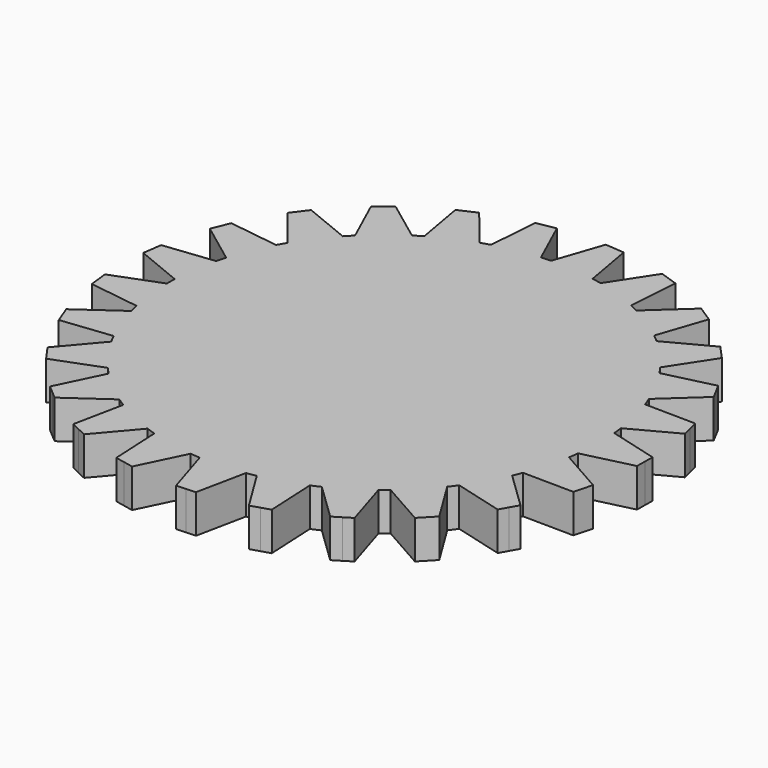
from build123d import *

# Parameters (mm, degrees)
F1_DEPTH = 4


# Not quite as in the source:
# - a feature names something its author has since deleted; it is built from what else it names


with BuildPart() as f1:
    # F0 (on Top) → F1 (new body)
    with BuildSketch(Plane.XY):
        with BuildLine():
            ThreePointArc((-15.8207142224, 15.9985937349), (-16.1763177404, 15.6389495927), (-16.5237476958, 15.2714034091))
            ThreePointArc((-16.5237476958, 15.2714034091), (-17.2896362976, 14.3985581465), (-18.0094723367, 13.4873609781))
            ThreePointArc((-18.0094723367, 13.4873609781), (-18.6807530995, 12.5411109411), (-19.3023658635, 11.5615168585))
            ThreePointArc((-19.3023658635, 11.5615168585), (-19.557357582, 11.1247365996), (-19.8024673676, 10.6823352389))
            ThreePointArc((-19.8024673676, 10.6823352389), (-20.7974411865, 8.585827863), (-21.5711788684, 6.3979873576))
            ThreePointArc((-21.5711788684, 6.3979873576), (-21.7095367198, 5.9115154921), (-21.8369251863, 5.4220566587))
            ThreePointArc((-21.8369251863, 5.4220566587), (-22.2792598903, 3.1439749905), (-22.4845953717, 0.8324487809))
            ThreePointArc((-22.4845953717, 0.8324487809), (-22.4976258234, 0.3268521252), (-22.4992886849, -0.1789096823))
            ThreePointArc((-22.4992886849, -0.1789096823), (-22.3611907578, -2.4954253934), (-21.9852220552, -4.7853956142))
            ThreePointArc((-21.9852220552, -4.7853956142), (-21.872106356, -5.2783485629), (-21.7479391288, -5.76863447))
            ThreePointArc((-21.7479391288, -5.76863447), (-21.0380857712, -7.9780290224), (-20.104436381, -10.1025560035))
            ThreePointArc((-20.104436381, -10.1025560035), (-19.8722820063, -10.5518911983), (-19.630086574, -10.9958947383))
            ThreePointArc((-19.630086574, -10.9958947383), (-18.393080483, -12.9593437467), (-16.96041503, -14.7849356444))
            ThreePointArc((-16.96041503, -14.7849356444), (-16.623809093, -15.1624197026), (-16.2788034853, -15.5322425002))
            ThreePointArc((-16.2788034853, -15.5322425002), (-14.5923703031, -17.1263752422), (-12.7507084267, -18.5383234036))
            ThreePointArc((-12.7507084267, -18.5383234036), (-12.3308011164, -18.8202376135), (-11.9046633044, -19.0926423422))
            ThreePointArc((-11.9046633044, -19.0926423422), (-9.87476783, -20.2172935949), (-7.7398279191, -21.1268801242))
            ThreePointArc((-7.7398279191, -21.1268801242), (-7.263003556, -21.2955107792), (-6.7825093458, -21.4533812481))
            ThreePointArc((-6.7825093458, -21.4533812481), (-4.5366973773, -22.0378850371), (-2.2426255582, -22.3879572674))
            ThreePointArc((-2.2426255582, -22.3879572674), (-1.7388447708, -22.4327086832), (-1.2341853806, -22.46612531))
            ThreePointArc((-1.2341853806, -22.46612531), (1.0864304565, -22.4737551126), (3.3954892143, -22.2423167183))
            ThreePointArc((3.3954892143, -22.2423167183), (3.8945720264, -22.1603769988), (4.391686991, -22.0672400942))
            ThreePointArc((4.391686991, -22.0672400942), (6.641293869, -21.4975165018), (8.8202529117, -20.6991096082))
            ThreePointArc((8.8202529117, -20.6991096082), (9.28327854, -20.4956273275), (9.7416135175, -20.2817890255))
            ThreePointArc((9.7416135175, -20.2817890255), (11.7788603628, -19.1705098668), (13.69080768, -17.8553013155))
            ThreePointArc((13.69080768, -17.8553013155), (14.0886825213, -17.5430620136), (14.4794386395, -17.2219585612))
            ThreePointArc((14.4794386395, -17.2219585612), (16.1763177404, -15.6389495927), (17.7011186506, -13.8895787739))
            ThreePointArc((17.7011186506, -13.8895787739), (18.0088427653, -13.4882015945), (18.3074673802, -13.0800091026))
            ThreePointArc((18.3074673802, -13.0800091026), (19.557357582, -11.1247365996), (20.5992032362, -9.0511229157))
            ThreePointArc((20.5992032362, -9.0511229157), (20.7974411865, -8.585827863), (20.9851706152, -8.1161945671))
            ThreePointArc((20.9851706152, -8.1161945671), (21.7095367198, -5.9115154921), (22.2029641238, -3.643951717))
            ThreePointArc((22.2029641238, -3.643951717), (22.2792598903, -3.1439749905), (22.3442984024, -2.6424096777))
            ThreePointArc((22.3442984024, -2.6424096777), (22.4610408714, -1.3234964953), (22.5, 0))
            ThreePointArc((22.5, 0), (22.4778969231, 0.9970706661), (22.4116311188, 1.9921823697))
            ThreePointArc((22.4116311188, 1.9921823697), (22.3611907578, 2.4954253934), (22.2994517444, 2.9974075298))
            ThreePointArc((22.2994517444, 2.9974075298), (21.872106356, 5.2783485629), (21.2120929064, 7.5031403113))
            ThreePointArc((21.2120929064, 7.5031403113), (21.0380857712, 7.9780290224), (20.8534485216, 8.4488865986))
            ThreePointArc((20.8534485216, 8.4488865986), (19.8722820063, 10.5518911983), (18.679720884, 12.5426483525))
            ThreePointArc((18.679720884, 12.5426483525), (18.393080483, 12.9593437467), (18.0971464347, 13.3694910495))
            ThreePointArc((18.0971464347, 13.3694910495), (16.623809093, 15.1624197026), (14.9736332993, 16.7940556691))
            ThreePointArc((14.9736332993, 16.7940556691), (14.5923703031, 17.1263752422), (14.2037340805, 17.4500412082))
            ThreePointArc((14.2037340805, 17.4500412082), (12.3308011164, 18.8202376135), (10.3266972653, 19.9902307038))
            ThreePointArc((10.3266972653, 19.9902307038), (9.87476783, 20.2172935949), (9.4178488765, 20.4341411011))
            ThreePointArc((9.4178488765, 20.4341411011), (7.263003556, 21.2955107792), (5.0308968631, 21.9303460245))
            ThreePointArc((5.0308968631, 21.9303460245), (4.5366973773, 22.0378850371), (4.0402055911, 22.1342887571))
            ThreePointArc((4.0402055911, 22.1342887571), (1.7388447708, 22.4327086832), (-0.5810132914, 22.4924970502))
            ThreePointArc((-0.5810132914, 22.4924970502), (-1.0864304565, 22.4737551126), (-1.5912986705, 22.4436576462))
            ThreePointArc((-1.5912986705, 22.4436576462), (-3.8945720264, 22.1603769988), (-6.1564162439, 21.6413617647))
            ThreePointArc((-6.1564162439, 21.6413617647), (-6.641293869, 21.4975165018), (-7.1228157842, 21.3428089835))
            ThreePointArc((-7.1228157842, 21.3428089835), (-9.28327854, 20.4956273275), (-11.3449889221, 19.4304201282))
            ThreePointArc((-11.3449889221, 19.4304201282), (-11.7788603628, 19.1705098668), (-12.2067801862, 18.9009131389))
            ThreePointArc((-12.2067801862, 18.9009131389), (-14.0886825213, 17.5430620136), (-15.8207142224, 15.9985937349))
        make_face()
        with BuildLine():
            ThreePointArc((-18.0094723367, 13.4873609781), (-17.2896362976, 14.3985581465), (-16.5237476958, 15.2714034091))
            Line((-16.5237476958, 15.2714034091), (-21.4175280286, 17.2801378501))
            Line((-21.4175280286, 17.2801378501), (-22.0158291312, 16.4788664912))
            Line((-22.0158291312, 16.4788664912), (-18.0094723367, 13.4873609781))
        make_face()
        with BuildLine():
            ThreePointArc((-19.3023658635, 11.5615168585), (-18.6807530995, 12.5411109411), (-18.0094723367, 13.4873609781))
            Line((-18.0094723367, 13.4873609781), (-22.0158291312, 16.4788664912))
            Line((-22.0158291312, 16.4788664912), (-22.6141302339, 15.6775951323))
            Line((-22.6141302339, 15.6775951323), (-19.3023658635, 11.5615168585))
        make_face()
        with BuildLine():
            Line((-18.0048063836, 20.8089601483), (-15.8207142224, 15.9985937349))
            ThreePointArc((-15.8207142224, 15.9985937349), (-14.0886825213, 17.5430620136), (-12.2067801862, 18.9009131389))
            Line((-12.2067801862, 18.9009131389), (-16.4472614694, 22.0635731724))
            Line((-16.4472614694, 22.0635731724), (-17.2260339265, 21.4362666603))
            Line((-17.2260339265, 21.4362666603), (-18.0048063836, 20.8089601483))
        make_face()
        with BuildLine():
            ThreePointArc((-21.5711788684, 6.3979873576), (-20.7974411865, 8.585827863), (-19.8024673676, 10.6823352389))
            Line((-19.8024673676, 10.6823352389), (-25.0420525337, 11.4109279148))
            Line((-25.0420525337, 11.4109279148), (-25.4222888231, 10.4860385354))
            Line((-25.4222888231, 10.4860385354), (-25.8025251126, 9.5611491559))
            Line((-25.8025251126, 9.5611491559), (-21.5711788684, 6.3979873576))
        make_face()
        with BuildLine():
            Line((-12.2641743313, 24.6328216682), (-11.3449889221, 19.4304201282))
            ThreePointArc((-11.3449889221, 19.4304201282), (-9.28327854, 20.4956273275), (-7.1228157842, 21.3428089835))
            Line((-7.1228157842, 21.3428089835), (-10.4435529833, 25.4606730481))
            Line((-10.4435529833, 25.4606730481), (-11.3538636573, 25.0467473581))
            Line((-11.3538636573, 25.0467473581), (-12.2641743313, 24.6328216682))
        make_face()
        with BuildLine():
            ThreePointArc((-22.4845953717, 0.8324487809), (-22.2792598903, 3.1439749905), (-21.8369251863, 5.4220566587))
            Line((-21.8369251863, 5.4220566587), (-27.0930927798, 4.8247274121))
            Line((-27.0930927798, 4.8247274121), (-27.2313726116, 3.8343342134))
            Line((-27.2313726116, 3.8343342134), (-27.3696524434, 2.8439410147))
            Line((-27.3696524434, 2.8439410147), (-22.4845953717, 0.8324487809))
        make_face()
        with BuildLine():
            Line((-5.7529391012, 26.9089124095), (-6.1564162439, 21.6413617647))
            ThreePointArc((-6.1564162439, 21.6413617647), (-3.8945720264, 22.1603769988), (-1.5912986705, 22.4436576462))
            Line((-1.5912986705, 22.4436576462), (-3.7836376545, 27.2579851984))
            Line((-3.7836376545, 27.2579851984), (-4.7682883778, 27.083448804))
            Line((-4.7682883778, 27.083448804), (-5.7529391012, 26.9089124095))
        make_face()
        with BuildLine():
            ThreePointArc((-21.9852220552, -4.7853956142), (-22.3611907578, -2.4954253934), (-22.4992886849, -0.1789096823))
            Line((-22.4992886849, -0.1789096823), (-27.4417743651, -2.0646284579))
            Line((-27.4417743651, -2.0646284579), (-27.3294091089, -3.0582954289))
            Line((-27.3294091089, -3.0582954289), (-27.2170438526, -4.0519623998))
            Line((-27.2170438526, -4.0519623998), (-21.9852220552, -4.7853956142))
        make_face()
        with BuildLine():
            Line((1.1197744504, 27.4942172201), (-0.5810132914, 22.4924970502))
            ThreePointArc((-0.5810132914, 22.4924970502), (1.7388447708, 22.4327086832), (4.0402055911, 22.1342887571))
            Line((4.0402055911, 22.1342887571), (3.1140175434, 27.3425778908))
            Line((3.1140175434, 27.3425778908), (2.1168959969, 27.4183975554))
            Line((2.1168959969, 27.4183975554), (1.1197744504, 27.4942172201))
        make_face()
        with BuildLine():
            ThreePointArc((-20.104436381, -10.1025560035), (-21.0380857712, -7.9780290224), (-21.7479391288, -5.76863447))
            Line((-21.7479391288, -5.76863447), (-26.0661883433, -8.8242561288))
            Line((-26.0661883433, -8.8242561288), (-25.7102383213, -9.7587611217))
            Line((-25.7102383213, -9.7587611217), (-25.3542882993, -10.6932661147))
            Line((-25.3542882993, -10.6932661147), (-20.104436381, -10.1025560035))
        make_face()
        with BuildLine():
            Line((7.9221284551, 26.3519592461), (5.0308968631, 21.9303460245))
            ThreePointArc((5.0308968631, 21.9303460245), (7.263003556, 21.2955107792), (9.4178488765, 20.4341411011))
            Line((9.4178488765, 20.4341411011), (9.8160075665, 25.7091358554))
            Line((9.8160075665, 25.7091358554), (8.8690680108, 26.0305475507))
            Line((8.8690680108, 26.0305475507), (7.9221284551, 26.3519592461))
        make_face()
        with BuildLine():
            ThreePointArc((-16.96041503, -14.7849356444), (-18.393080483, -12.9593437467), (-19.630086574, -10.9958947383))
            Line((-19.630086574, -10.9958947383), (-23.0527678432, -15.0294233337))
            Line((-23.0527678432, -15.0294233337), (-22.4755987044, -15.8460479631))
            Line((-22.4755987044, -15.8460479631), (-21.8984295657, -16.6626725925))
            Line((-21.8984295657, -16.6626725925), (-16.96041503, -14.7849356444))
        make_face()
        with BuildLine():
            Line((14.2267059934, 23.5539107569), (10.3266972653, 19.9902307038))
            ThreePointArc((10.3266972653, 19.9902307038), (12.3308011164, 18.8202376135), (14.2037340805, 17.4500412082))
            Line((14.2037340805, 17.4500412082), (15.9012217334, 22.4602942626))
            Line((15.9012217334, 22.4602942626), (15.0639638634, 23.0071025097))
            Line((15.0639638634, 23.0071025097), (14.2267059934, 23.5539107569))
        make_face()
        with BuildLine():
            ThreePointArc((-12.7507084267, -18.5383234036), (-14.5923703031, -17.1263752422), (-16.2788034853, -15.5322425002))
            Line((-16.2788034853, -15.5322425002), (-18.5908571573, -20.2902365963))
            Line((-18.5908571573, -20.2902365963), (-17.8287345614, -20.9376693333))
            Line((-17.8287345614, -20.9376693333), (-17.0666119656, -21.5851020702))
            Line((-17.0666119656, -21.5851020702), (-12.7507084267, -18.5383234036))
        make_face()
        with BuildLine():
            Line((19.637367272, 19.2758834296), (14.9736332993, 16.7940556691))
            ThreePointArc((14.9736332993, 16.7940556691), (16.623809093, 15.1624197026), (18.0971464347, 13.3694910495))
            Line((18.0971464347, 13.3694910495), (20.9873036582, 17.8001897781))
            Line((20.9873036582, 17.8001897781), (20.3123354651, 18.5380366038))
            Line((20.3123354651, 18.5380366038), (19.637367272, 19.2758834296))
        make_face()
        with BuildLine():
            ThreePointArc((-7.7398279191, -21.1268801242), (-9.87476783, -20.2172935949), (-11.9046633044, -19.0926423422))
            Line((-11.9046633044, -19.0926423422), (-12.9608145438, -24.2761396712))
            Line((-12.9608145438, -24.2761396712), (-12.0616254564, -24.7136999358))
            Line((-12.0616254564, -24.7136999358), (-11.1624363691, -25.1512602005))
            Line((-11.1624363691, -25.1512602005), (-7.7398279191, -21.1268801242))
        make_face()
        with BuildLine():
            Line((23.8141405436, 13.7866814547), (18.679720884, 12.5426483525))
            ThreePointArc((18.679720884, 12.5426483525), (19.8722820063, 10.5518911983), (20.8534485216, 8.4488865986))
            Line((20.8534485216, 8.4488865986), (24.7546761082, 12.0216339053))
            Line((24.7546761082, 12.0216339053), (24.2844083259, 12.90415768))
            Line((24.2844083259, 12.90415768), (23.8141405436, 13.7866814547))
        make_face()
        with BuildLine():
            ThreePointArc((-2.2426255582, -22.3879572674), (-4.5366973773, -22.0378850371), (-6.7825093458, -21.4533812481))
            Line((-6.7825093458, -21.4533812481), (-6.516396286, -26.7366836092))
            Line((-6.516396286, -26.7366836092), (-5.5366400645, -26.9368778808))
            Line((-5.5366400645, -26.9368778808), (-4.556883843, -27.1370721525))
            Line((-4.556883843, -27.1370721525), (-2.2426255582, -22.3879572674))
        make_face()
        with BuildLine():
            Line((26.4945837827, 7.4312115802), (21.2120929064, 7.5031403113))
            ThreePointArc((21.2120929064, 7.5031403113), (21.872106356, 5.2783485629), (22.2994517444, 2.9974075298))
            Line((22.2994517444, 2.9974075298), (26.966621217, 5.4877145618))
            Line((26.966621217, 5.4877145618), (26.7306024999, 6.459463071))
            Line((26.7306024999, 6.459463071), (26.4945837827, 7.4312115802))
        make_face()
        with BuildLine():
            ThreePointArc((3.3954892143, -22.2423167183), (1.0864304565, -22.4737551126), (-1.2341853806, -22.46612531))
            Line((-1.2341853806, -22.46612531), (0.3374711161, -27.5172633854))
            Line((0.3374711161, -27.5172633854), (1.3362327851, -27.4675127217))
            Line((1.3362327851, -27.4675127217), (2.3349944541, -27.4177620579))
            Line((2.3349944541, -27.4177620579), (3.3954892143, -22.2423167183))
        make_face()
        with BuildLine():
            Line((27.5102748824, 0.608811352), (22.4116311188, 1.9921823697))
            ThreePointArc((22.4116311188, 1.9921823697), (22.4778969231, 0.9970706661), (22.5, 0))
            ThreePointArc((22.5, 0), (22.4610408714, -1.3234964953), (22.3442984024, -2.6424096777))
            Line((22.3442984024, -2.6424096777), (27.4841543385, -1.3910180701))
            Line((27.4841543385, -1.3910180701), (27.4972146104, -0.3911033591))
            Line((27.4972146104, -0.3911033591), (27.5102748824, 0.608811352))
        make_face()
        with BuildLine():
            ThreePointArc((8.8202529117, -20.6991096082), (6.641293869, -21.4975165018), (4.391686991, -22.0672400942))
            Line((4.391686991, -22.0672400942), (7.1701339668, -26.5688323017))
            Line((7.1701339668, -26.5688323017), (8.1251452144, -26.2722627197))
            Line((8.1251452144, -26.2722627197), (9.080156462, -25.9756931378))
            Line((9.080156462, -25.9756931378), (8.8202529117, -20.6991096082))
        make_face()
        with BuildLine():
            Line((26.7973942355, -6.2518427326), (22.2029641238, -3.643951717))
            ThreePointArc((22.2029641238, -3.643951717), (21.7095367198, -5.9115154921), (20.9851706152, -8.1161945671))
            Line((20.9851706152, -8.1161945671), (26.2747569633, -8.1823479208))
            Line((26.2747569633, -8.1823479208), (26.5360755994, -7.2170953267))
            Line((26.5360755994, -7.2170953267), (26.7973942355, -6.2518427326))
        make_face()
        with BuildLine():
            ThreePointArc((13.69080768, -17.8553013155), (11.7788603628, -19.1705098668), (9.7416135175, -20.2817890255))
            Line((9.7416135175, -20.2817890255), (13.5522709305, -23.9509837711))
            Line((13.5522709305, -23.9509837711), (14.4035248878, -23.4262298285))
            Line((14.4035248878, -23.4262298285), (15.254778845, -22.901475886))
            Line((15.254778845, -22.901475886), (13.69080768, -17.8553013155))
        make_face()
        with BuildLine():
            Line((24.4007347549, -12.7196705455), (20.5992032362, -9.0511229157))
            ThreePointArc((20.5992032362, -9.0511229157), (19.557357582, -11.1247365996), (18.3074673802, -13.0800091026))
            Line((18.3074673802, -13.0800091026), (23.4144199762, -14.459550759))
            Line((23.4144199762, -14.459550759), (23.9075773656, -13.5896106523))
            Line((23.9075773656, -13.5896106523), (24.4007347549, -12.7196705455))
        make_face()
        with BuildLine():
            ThreePointArc((17.7011186506, -13.8895787739), (16.1763177404, -15.6389495927), (14.4794386395, -17.2219585612))
            Line((14.4794386395, -17.2219585612), (19.0828688698, -19.8282068446))
            Line((19.0828688698, -19.8282068446), (19.7768781199, -19.1082407615))
            Line((19.7768781199, -19.1082407615), (20.47088737, -18.3882746784))
            Line((20.47088737, -18.3882746784), (17.7011186506, -13.8895787739))
        make_face()
    extrude(amount=F1_DEPTH)


solid = f1.part
